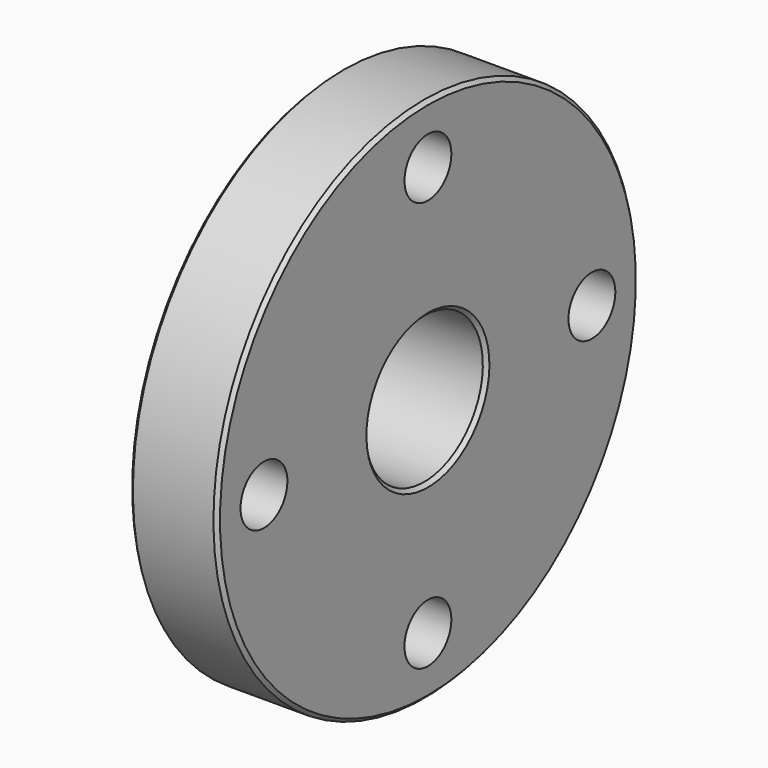
from build123d import *

# Parameters (mm, degrees)
F2_SIZE         = 0.5
F3_R            = 4
F4_DEPTH        = 18.001
F4_COPIES_COUNT = 4


# Not quite as in the source:
# - a pattern or mirror of a feature is missing from the dataset's text; its kind, count and spacing are read off the source's solid


with BuildPart() as f1:
    # F0 (on Front) → F1 (revolve)
    with BuildSketch(Plane.XZ):
        Polygon((-18, 10), (0, 10), (0, 36), (-12, 36), (-12, 20), (-18, 20), align=None)
    revolve(axis=Axis((-9, 0, 0), (1, 0, 0)))

    # F2
    f2_edges = [f1.edges().sort_by_distance(p)[0] for p in [
        (-18, 0, -20),
        (-18, 0, -10),
        (-12, 0, -36),
        (0, 0, -10),
        (0, 0, -36),
    ]]
    chamfer(f2_edges, length=F2_SIZE)

    # F3 (on Right) → F4 (cut, through all)
    with BuildSketch(Plane.YZ):
        with Locations((0, 28)):
            Circle(F3_R)
    f4 = extrude(amount=-F4_DEPTH, mode=Mode.SUBTRACT)

    # F4_copies: F4 ×4 about axis
    f4_copies_axis = Axis((0, 0, 0), (1, 0, 0))
    for i in range(1, F4_COPIES_COUNT):
        add(f4.rotate(f4_copies_axis, i * 360 / F4_COPIES_COUNT), mode=Mode.SUBTRACT)


solid = f1.part
